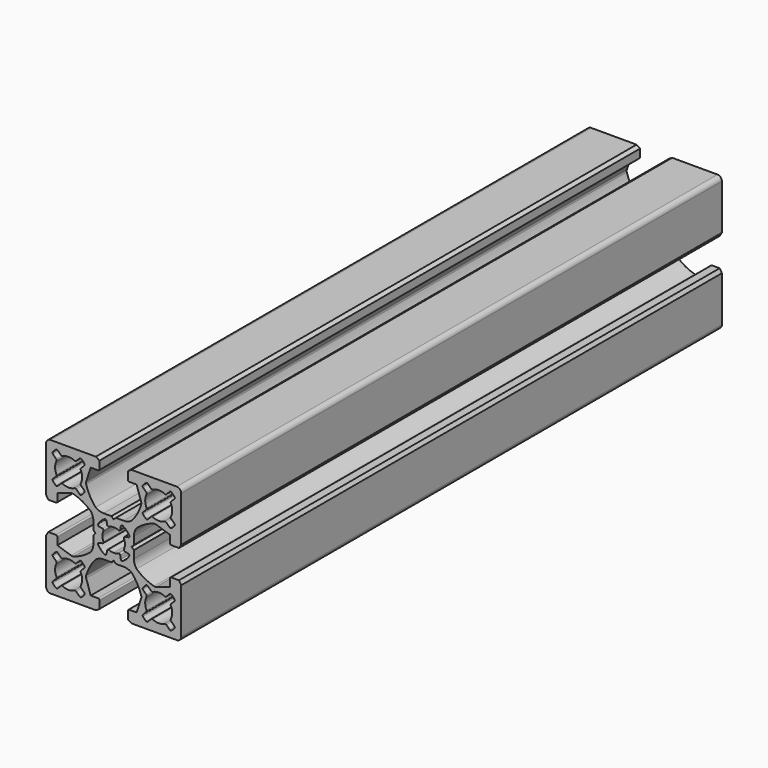
from build123d import *

# Parameters (mm, degrees)
F1_DEPTH = 150


# Not quite as in the source:
# - ends of sketch curves that miss each other by under 0.0002 mm in the source are joined


with BuildPart() as f1:
    # F0 (on Front) → F1 (new body)
    with BuildSketch(Plane.XZ):
        with BuildLine():
            Line((-10.317882, -28.053804), (-8.817882, -28.053804))
            Line((-8.817882, -28.053804), (-8.317882, -27.553804))
            Line((-8.317882, -27.553804), (-8.317882, -25.835963))
            ThreePointArc((-8.317882, -25.835963), (-8.1666472628, -24.8954650055), (-7.7281910149, -24.049790989))
            ThreePointArc((-7.7281910149, -24.049790989), (-5.9278016138, -22.7791417483), (-3.8900220756, -21.9404487353))
            ThreePointArc((-3.8900220756, -21.9404487353), (-3.6281322729, -21.9188378518), (-3.3696549943, -21.9661959825))
            Line((-3.3696549943, -21.9661959825), (-0.317882, -22.953804))
            Line((-0.317882, -22.953804), (-0.317882, -24.603804))
            ThreePointArc((-0.317882, -24.603804), (-0.2300140344, -24.8159360344), (-0.017882, -24.903804))
            Line((-0.017882, -24.903804), (1.682118, -24.903804))
            Line((1.682118, -24.903804), (2.182118, -24.103804))
            Line((2.182118, -24.103804), (2.182118, -14.053804))
            ThreePointArc((2.182118, -14.053804), (1.8892247812, -13.3466972188), (1.182118, -13.053804))
            Line((1.182118, -13.053804), (-8.867882, -13.053804))
            Line((-8.867882, -13.053804), (-9.667882, -13.553804))
            Line((-9.667882, -13.553804), (-9.667882, -15.253804))
            ThreePointArc((-9.667882, -15.253804), (-9.5800140344, -15.4659360344), (-9.367882, -15.553804))
            Line((-9.367882, -15.553804), (-7.717882, -15.553804))
            Line((-7.717882, -15.553804), (-6.730274, -18.605577))
            ThreePointArc((-6.730274, -18.605577), (-6.6829159047, -18.8640542036), (-6.7045263914, -19.1259439149))
            ThreePointArc((-6.7045263914, -19.1259439149), (-7.5432189083, -21.1637239049), (-8.8138685119, -22.9641134339))
            ThreePointArc((-8.8138685119, -22.9641134339), (-9.6595430055, -23.4025692628), (-10.600041, -23.553804))
            Line((-10.600041, -23.553804), (-12.317882, -23.553804))
            Line((-12.317882, -23.553804), (-12.817882, -24.053804))
            Line((-12.817882, -24.053804), (-12.817882, -25.553804))
            ThreePointArc((-12.817882, -25.553804), (-12.2892723342, -25.6103286428), (-11.7845662465, -25.777346543))
            ThreePointArc((-11.7845662465, -25.777346543), (-11.521192295, -25.7698304515), (-11.3653270693, -25.5573959875))
            Line((-11.3653270693, -25.5573959875), (-11.231756, -24.816462))
            ThreePointArc((-11.231756, -24.816462), (-11.061392872, -24.5969122529), (-10.7838767336, -24.6114195492))
            ThreePointArc((-10.7838767336, -24.6114195492), (-9.990624391, -25.2265473595), (-9.3754974572, -26.0198002702))
            ThreePointArc((-9.3754974572, -26.0198002702), (-9.3609903588, -26.2973161033), (-9.5805400125, -26.4676789307))
            Line((-9.5805400125, -26.4676789307), (-10.321473, -26.601249))
            ThreePointArc((-10.321473, -26.601249), (-10.5339073555, -26.757114112), (-10.5414238716, -27.0204879417))
            ThreePointArc((-10.5414238716, -27.0204879417), (-10.3744066428, -27.5251943342), (-10.317882, -28.053804))
        make_face()
        with BuildLine():
            ThreePointArc((-5.5627339656, -19.7356560344), (-5.4787894201, -19.5718836819), (-5.5062620121, -19.389913006))
            ThreePointArc((-5.5062620121, -19.389913006), (-5.820221, -18.053804), (-5.5062614757, -16.7176952608))
            ThreePointArc((-5.5062614757, -16.7176952608), (-5.4787894201, -16.5357243181), (-5.5627339656, -16.3719519656))
            Line((-5.5627339656, -16.3719519656), (-6.303305, -15.631381))
            ThreePointArc((-6.303305, -15.631381), (-6.3907399595, -15.4353436467), (-6.3248118511, -15.2310671199))
            ThreePointArc((-6.3248118511, -15.2310671199), (-6.0022020125, -14.8718239818), (-5.6429589383, -14.5492140766))
            ThreePointArc((-5.6429589383, -14.5492140766), (-5.4386817022, -14.4832850218), (-5.2426439656, -14.5707209656))
            Line((-5.2426439656, -14.5707209656), (-4.502074, -15.311292))
            ThreePointArc((-4.502074, -15.311292), (-4.3383016819, -15.3952365799), (-4.156331006, -15.3677639879))
            ThreePointArc((-4.156331006, -15.3677639879), (-2.8202214477, -15.053804), (-1.484111862, -15.3677637227))
            ThreePointArc((-1.484111862, -15.3677637227), (-1.3021413181, -15.3952365799), (-1.1383689656, -15.3112920344))
            Line((-1.1383689656, -15.3112920344), (-0.397799, -14.570721))
            ThreePointArc((-0.397799, -14.570721), (-0.2017612978, -14.4832850218), (0.0025159751, -14.5492140309))
            ThreePointArc((0.0025159751, -14.5492140309), (0.3617595153, -14.8718234847), (0.684369412, -15.2310666682))
            ThreePointArc((0.684369412, -15.2310666682), (0.7502979573, -15.4353436866), (0.6628620344, -15.6313810344))
            Line((0.6628620344, -15.6313810344), (-0.077709, -16.371952))
            ThreePointArc((-0.077709, -16.371952), (-0.1616535799, -16.5357243181), (-0.1341809879, -16.717694994))
            ThreePointArc((-0.1341809879, -16.717694994), (0.179779, -18.053804), (-0.1341807227, -19.389913138))
            ThreePointArc((-0.1341807227, -19.389913138), (-0.1616535799, -19.5718836819), (-0.0777090344, -19.7356560344))
            Line((-0.0777090344, -19.7356560344), (0.662862, -20.476227))
            ThreePointArc((0.662862, -20.476227), (0.7502979573, -20.6722643134), (0.6843694576, -20.8765413686))
            ThreePointArc((0.6843694576, -20.8765413686), (0.3617595153, -21.2357845153), (0.0025163318, -21.558394412))
            ThreePointArc((0.0025163318, -21.558394412), (-0.2017612978, -21.6243229782), (-0.3977990344, -21.5368870344))
            Line((-0.3977990344, -21.5368870344), (-1.138369, -20.796316))
            ThreePointArc((-1.138369, -20.796316), (-1.3021413181, -20.7123714201), (-1.484111994, -20.7398440121))
            ThreePointArc((-1.484111994, -20.7398440121), (-2.8202214477, -21.053804), (-4.1563309396, -20.7398438786))
            ThreePointArc((-4.1563309396, -20.7398438786), (-4.3383016819, -20.7123714201), (-4.5020740344, -20.7963159656))
            Line((-4.5020740344, -20.7963159656), (-5.242644, -21.536887))
            ThreePointArc((-5.242644, -21.536887), (-5.4386817022, -21.6243229782), (-5.6429589751, -21.5583939691))
            ThreePointArc((-5.6429589751, -21.5583939691), (-6.0022020125, -21.2357840182), (-6.3248118054, -20.8765408433))
            ThreePointArc((-6.3248118054, -20.8765408433), (-6.3907399595, -20.6722643533), (-6.3033045344, -20.4762274656))
            Line((-6.3033045344, -20.4762274656), (-5.5627339656, -19.7356560344))
        make_face(mode=Mode.SUBTRACT)
        with BuildLine():
            Line((-16.817882, -28.053804), (-15.317882, -28.053804))
            ThreePointArc((-15.317882, -28.053804), (-15.2613573135, -27.5251941322), (-15.0943392862, -27.0204878701))
            ThreePointArc((-15.0943392862, -27.0204878701), (-15.1018556445, -26.757114112), (-15.3142900125, -26.6012490693))
            Line((-15.3142900125, -26.6012490693), (-16.055223, -26.467679))
            ThreePointArc((-16.055223, -26.467679), (-16.2747726412, -26.2973161033), (-16.2602657097, -26.0198001716))
            ThreePointArc((-16.2602657097, -26.0198001716), (-15.6451391247, -25.2265468753), (-14.8518861678, -24.611419716))
            ThreePointArc((-14.8518861678, -24.611419716), (-14.574370128, -24.5969122529), (-14.4040070693, -24.8164620125))
            Line((-14.4040070693, -24.8164620125), (-14.270436, -25.557396))
            ThreePointArc((-14.270436, -25.557396), (-14.114570705, -25.7698304515), (-13.8511966819, -25.7773467007))
            ThreePointArc((-13.8511966819, -25.7773467007), (-13.3464912208, -25.6103285465), (-12.817882, -25.553804))
            Line((-12.817882, -25.553804), (-12.817882, -24.053804))
            Line((-12.817882, -24.053804), (-13.317882, -23.553804))
            Line((-13.317882, -23.553804), (-15.035723, -23.553804))
            ThreePointArc((-15.035723, -23.553804), (-15.9762206131, -23.4025693887), (-16.8218943655, -22.9641134932))
            ThreePointArc((-16.8218943655, -22.9641134932), (-18.0925440917, -21.1637239049), (-18.9312372647, -19.1259440756))
            ThreePointArc((-18.9312372647, -19.1259440756), (-18.952848093, -18.864054156), (-18.9054896298, -18.6055767962))
            Line((-18.9054896298, -18.6055767962), (-17.917882, -15.553804))
            Line((-17.917882, -15.553804), (-16.267882, -15.553804))
            ThreePointArc((-16.267882, -15.553804), (-16.0557499656, -15.4659360344), (-15.967882, -15.253804))
            Line((-15.967882, -15.253804), (-15.967882, -13.553804))
            Line((-15.967882, -13.553804), (-16.767882, -13.053804))
            Line((-16.767882, -13.053804), (-26.817882, -13.053804))
            ThreePointArc((-26.817882, -13.053804), (-27.5249887812, -13.3466972188), (-27.817882, -14.053804))
            Line((-27.817882, -14.053804), (-27.817882, -24.103804))
            Line((-27.817882, -24.103804), (-27.317882, -24.903804))
            Line((-27.317882, -24.903804), (-25.617882, -24.903804))
            ThreePointArc((-25.617882, -24.903804), (-25.4057499656, -24.8159360344), (-25.317882, -24.603804))
            Line((-25.317882, -24.603804), (-25.317882, -22.953804))
            Line((-25.317882, -22.953804), (-22.266108, -21.966196))
            ThreePointArc((-22.266108, -21.966196), (-22.0076307271, -21.9188378518), (-21.7457409226, -21.9404486442))
            ThreePointArc((-21.7457409226, -21.9404486442), (-19.7079616374, -22.7791421598), (-17.907572504, -24.049791567))
            ThreePointArc((-17.907572504, -24.049791567), (-17.4691166439, -24.8954652882), (-17.317882, -25.835963))
            Line((-17.317882, -25.835963), (-17.317882, -27.553804))
            Line((-17.317882, -27.553804), (-16.817882, -28.053804))
        make_face()
        with BuildLine():
            ThreePointArc((-20.1318415243, -16.7176952608), (-19.817882, -18.053804), (-20.1318415243, -19.3899127392))
            ThreePointArc((-20.1318415243, -19.3899127392), (-20.1593135799, -19.5718836819), (-20.0753690344, -19.7356560344))
            Line((-20.0753690344, -19.7356560344), (-19.334799, -20.476227))
            ThreePointArc((-19.334799, -20.476227), (-19.2473630595, -20.6722640002), (-19.3132911489, -20.8765408801))
            ThreePointArc((-19.3132911489, -20.8765408801), (-19.6359009875, -21.2357840182), (-19.9951440617, -21.5583939234))
            ThreePointArc((-19.9951440617, -21.5583939234), (-20.1994212978, -21.6243229782), (-20.3954590344, -21.5368870344))
            Line((-20.3954590344, -21.5368870344), (-21.136029, -20.796316))
            ThreePointArc((-21.136029, -20.796316), (-21.2998015274, -20.7123715492), (-21.4817721923, -20.7398436134))
            ThreePointArc((-21.4817721923, -20.7398436134), (-22.8178815523, -21.053804), (-24.153991138, -20.7398442773))
            ThreePointArc((-24.153991138, -20.7398442773), (-24.3359616819, -20.7123714201), (-24.4997340344, -20.7963159656))
            Line((-24.4997340344, -20.7963159656), (-25.240304, -21.536887))
            ThreePointArc((-25.240304, -21.536887), (-25.4363417022, -21.6243229782), (-25.6406189751, -21.5583939691))
            ThreePointArc((-25.6406189751, -21.5583939691), (-25.9998625153, -21.2357845153), (-26.322472412, -20.8765413318))
            ThreePointArc((-26.322472412, -20.8765413318), (-26.3884009573, -20.6722643134), (-26.3009650344, -20.4762269656))
            Line((-26.3009650344, -20.4762269656), (-25.560394, -19.735656))
            ThreePointArc((-25.560394, -19.735656), (-25.4764494201, -19.5718836819), (-25.5039220121, -19.389913006))
            ThreePointArc((-25.5039220121, -19.389913006), (-25.817882, -18.053804), (-25.5039222773, -16.717694862))
            ThreePointArc((-25.5039222773, -16.717694862), (-25.4764494201, -16.5357243181), (-25.5603939656, -16.3719519656))
            Line((-25.5603939656, -16.3719519656), (-26.300965, -15.631381))
            ThreePointArc((-26.300965, -15.631381), (-26.3884009573, -15.4353436866), (-26.3224724576, -15.2310666314))
            ThreePointArc((-26.3224724576, -15.2310666314), (-25.9998625153, -14.8718234847), (-25.6406193318, -14.549213588))
            ThreePointArc((-25.6406193318, -14.549213588), (-25.4363417022, -14.4832850218), (-25.2403039656, -14.5707209656))
            Line((-25.2403039656, -14.5707209656), (-24.499734, -15.311292))
            ThreePointArc((-24.499734, -15.311292), (-24.3359616819, -15.3952365799), (-24.153991006, -15.3677639879))
            ThreePointArc((-24.153991006, -15.3677639879), (-22.8178815523, -15.053804), (-21.4817720604, -15.3677641214))
            ThreePointArc((-21.4817720604, -15.3677641214), (-21.2998015274, -15.3952364508), (-21.1360294656, -15.3112915344))
            Line((-21.1360294656, -15.3112915344), (-20.395459, -14.570721))
            ThreePointArc((-20.395459, -14.570721), (-20.1994212978, -14.4832850218), (-19.9951440249, -14.5492140309))
            ThreePointArc((-19.9951440249, -14.5492140309), (-19.6359009875, -14.8718239818), (-19.3132911946, -15.2310671567))
            ThreePointArc((-19.3132911946, -15.2310671567), (-19.2473630595, -15.4353439998), (-19.3347989656, -15.6313810344))
            Line((-19.3347989656, -15.6313810344), (-20.075369, -16.371952))
            ThreePointArc((-20.075369, -16.371952), (-20.1593135799, -16.5357243181), (-20.1318415243, -16.7176952608))
        make_face(mode=Mode.SUBTRACT)
        with BuildLine():
            ThreePointArc((-15.0943392862, -29.0871201299), (-15.2613573135, -28.5824138678), (-15.317882, -28.053804))
            Line((-15.317882, -28.053804), (-16.817882, -28.053804))
            Line((-16.817882, -28.053804), (-17.317882, -28.553804))
            Line((-17.317882, -28.553804), (-17.317882, -30.271645))
            ThreePointArc((-17.317882, -30.271645), (-17.4691166439, -31.2121427118), (-17.9075726307, -32.0578165326))
            ThreePointArc((-17.9075726307, -32.0578165326), (-19.7079616374, -33.3284658402), (-21.7457409999, -34.1671590005))
            ThreePointArc((-21.7457409999, -34.1671590005), (-22.0076307271, -34.1887701482), (-22.2661080057, -34.1414120175))
            Line((-22.2661080057, -34.1414120175), (-25.317882, -33.153804))
            Line((-25.317882, -33.153804), (-25.317882, -31.503804))
            ThreePointArc((-25.317882, -31.503804), (-25.4057499656, -31.2916719656), (-25.617882, -31.203804))
            Line((-25.617882, -31.203804), (-27.317882, -31.203804))
            Line((-27.317882, -31.203804), (-27.817882, -32.003804))
            Line((-27.817882, -32.003804), (-27.817882, -42.053804))
            ThreePointArc((-27.817882, -42.053804), (-27.5249887812, -42.7609107812), (-26.817882, -43.053804))
            Line((-26.817882, -43.053804), (-16.767882, -43.053804))
            Line((-16.767882, -43.053804), (-15.967882, -42.553804))
            Line((-15.967882, -42.553804), (-15.967882, -40.853804))
            ThreePointArc((-15.967882, -40.853804), (-16.0557499656, -40.6416719656), (-16.267882, -40.553804))
            Line((-16.267882, -40.553804), (-17.917882, -40.553804))
            Line((-17.917882, -40.553804), (-18.905489, -37.50203))
            ThreePointArc((-18.905489, -37.50203), (-18.9528481165, -37.2435533689), (-18.9312375634, -36.9816638775))
            ThreePointArc((-18.9312375634, -36.9816638775), (-18.0925440917, -34.9438840951), (-16.8218944881, -33.1434945661))
            ThreePointArc((-16.8218944881, -33.1434945661), (-15.9762206131, -32.7050386113), (-15.035723, -32.553804))
            Line((-15.035723, -32.553804), (-13.317882, -32.553804))
            Line((-13.317882, -32.553804), (-12.817882, -32.053804))
            Line((-12.817882, -32.053804), (-12.817882, -30.553804))
            ThreePointArc((-12.817882, -30.553804), (-13.3464914228, -30.4972794098), (-13.8511973007, -30.3302616625))
            ThreePointArc((-13.8511973007, -30.3302616625), (-14.114570888, -30.3377776445), (-14.2704359307, -30.5502120125))
            Line((-14.2704359307, -30.5502120125), (-14.404007, -31.291146))
            ThreePointArc((-14.404007, -31.291146), (-14.574370128, -31.5106957471), (-14.8518862664, -31.4961884508))
            ThreePointArc((-14.8518862664, -31.4961884508), (-15.6451391247, -30.8810611247), (-16.260266284, -30.0878081678))
            ThreePointArc((-16.260266284, -30.0878081678), (-16.2747726412, -29.8102918967), (-16.0552229875, -29.6399290693))
            Line((-16.0552229875, -29.6399290693), (-15.31429, -29.506358))
            ThreePointArc((-15.31429, -29.506358), (-15.1018556033, -29.3504938095), (-15.0943392862, -29.0871201299))
        make_face()
        with BuildLine():
            ThreePointArc((-20.0747205338, -36.3725174663), (-20.1586523342, -36.5362963089), (-20.1311656295, -36.7182648157))
            ThreePointArc((-20.1311656295, -36.7182648157), (-19.8171020091, -38.0543498837), (-20.1309575628, -39.3904837201))
            ThreePointArc((-20.1309575628, -39.3904837201), (-20.1584156946, -39.5724564631), (-20.0744580337, -39.7362220337))
            Line((-20.0744580337, -39.7362220337), (-19.33383, -40.476735))
            ThreePointArc((-19.33383, -40.476735), (-19.2463783169, -40.6727656131), (-19.3122908476, -40.8770481227))
            ThreePointArc((-19.3122908476, -40.8770481227), (-19.6348730769, -41.2363160882), (-19.9940910142, -41.5589539824))
            ThreePointArc((-19.9940910142, -41.5589539824), (-20.1983629105, -41.6248982338), (-20.3944070337, -41.5374780337))
            Line((-20.3944070337, -41.5374780337), (-21.135036, -40.796965))
            ThreePointArc((-21.135036, -40.796965), (-21.2988146578, -40.7130336089), (-21.4807828157, -40.7405203705))
            ThreePointArc((-21.4807828157, -40.7405203705), (-22.8168676587, -41.0545839908), (-24.1530013171, -40.7407286377))
            ThreePointArc((-24.1530013171, -40.7407286377), (-24.334973892, -40.7132702121), (-24.4987395337, -40.7972274662))
            Line((-24.4987395337, -40.7972274662), (-25.239253, -41.537856))
            ThreePointArc((-25.239253, -41.537856), (-25.435283708, -41.625306742), (-25.6395657293, -41.5593936639))
            ThreePointArc((-25.6395657293, -41.5593936639), (-25.99883431, -41.2368127014), (-26.3214719824, -40.8775949858))
            ThreePointArc((-26.3214719824, -40.8775949858), (-26.3874162149, -40.6733227364), (-26.2999955337, -40.4772784662))
            Line((-26.2999955337, -40.4772784662), (-25.559483, -39.73665))
            ThreePointArc((-25.559483, -39.73665), (-25.475550759, -39.5728712621), (-25.5030371701, -39.3909025871))
            ThreePointArc((-25.5030371701, -39.3909025871), (-25.8171019909, -38.0548178936), (-25.503246239, -36.7186838812))
            ThreePointArc((-25.503246239, -36.7186838812), (-25.4757871762, -36.5367113277), (-25.5597444663, -36.3729454662))
            Line((-25.5597444663, -36.3729454662), (-26.300374, -35.632433))
            ThreePointArc((-26.300374, -35.632433), (-26.3878247021, -35.4364020339), (-26.3219121524, -35.2321198773))
            ThreePointArc((-26.3219121524, -35.2321198773), (-25.9993304261, -34.8728514147), (-25.6401123794, -34.550213529))
            ThreePointArc((-25.6401123794, -34.550213529), (-25.4358403078, -34.4842688081), (-25.2397959662, -34.5716899662))
            Line((-25.2397959662, -34.5716899662), (-24.499168, -35.312203))
            ThreePointArc((-24.499168, -35.312203), (-24.3353886912, -35.3961343342), (-24.1534201843, -35.3686476295))
            ThreePointArc((-24.1534201843, -35.3686476295), (-22.8173356686, -35.0545840091), (-21.4812022799, -35.3684395628))
            ThreePointArc((-21.4812022799, -35.3684395628), (-21.2992289788, -35.3958977668), (-21.1354629663, -35.3119400337))
            Line((-21.1354629663, -35.3119400337), (-20.39495, -34.571312))
            ThreePointArc((-20.39495, -34.571312), (-20.1989200339, -34.4838602979), (-19.9946378773, -34.5497728476))
            ThreePointArc((-19.9946378773, -34.5497728476), (-19.63536969, -34.8723552987), (-19.312731624, -35.2315735027))
            ThreePointArc((-19.312731624, -35.2315735027), (-19.2467867662, -35.4358449105), (-19.3342069663, -35.6318890337))
            Line((-19.3342069663, -35.6318890337), (-20.0747205338, -36.3725174663))
        make_face(mode=Mode.SUBTRACT)
        with BuildLine():
            Line((-8.317882, -28.553804), (-8.817882, -28.053804))
            Line((-8.817882, -28.053804), (-10.317882, -28.053804))
            ThreePointArc((-10.317882, -28.053804), (-10.3744066428, -28.5824136658), (-10.541424543, -29.0871197535))
            ThreePointArc((-10.541424543, -29.0871197535), (-10.5339073967, -29.3504938095), (-10.3214731621, -29.5063588992))
            Line((-10.3214731621, -29.5063588992), (-9.58054, -29.639929))
            ThreePointArc((-9.58054, -29.639929), (-9.3609903588, -29.8102918967), (-9.3754972903, -30.0878078284))
            ThreePointArc((-9.3754972903, -30.0878078284), (-9.990624391, -30.8810606405), (-10.783877091, -31.496187846))
            ThreePointArc((-10.783877091, -31.496187846), (-11.061392872, -31.5106957471), (-11.2317559307, -31.2911459875))
            Line((-11.2317559307, -31.2911459875), (-11.365327, -30.550212))
            ThreePointArc((-11.365327, -30.550212), (-11.521192112, -30.3377776445), (-11.7845659417, -30.3302611284))
            ThreePointArc((-11.7845659417, -30.3302611284), (-12.2892721322, -30.4972793135), (-12.817882, -30.553804))
            Line((-12.817882, -30.553804), (-12.817882, -32.053804))
            Line((-12.817882, -32.053804), (-12.317882, -32.553804))
            Line((-12.317882, -32.553804), (-10.600041, -32.553804))
            ThreePointArc((-10.600041, -32.553804), (-9.6595430055, -32.7050387372), (-8.813868989, -33.1434949851))
            ThreePointArc((-8.813868989, -33.1434949851), (-7.5432189083, -34.9438840951), (-6.7045257353, -36.9816639244))
            ThreePointArc((-6.7045257353, -36.9816639244), (-6.6829158812, -37.2435533212), (-6.7302739825, -37.5020300057))
            Line((-6.7302739825, -37.5020300057), (-7.717882, -40.553804))
            Line((-7.717882, -40.553804), (-9.367882, -40.553804))
            ThreePointArc((-9.367882, -40.553804), (-9.5800140344, -40.6416719656), (-9.667882, -40.853804))
            Line((-9.667882, -40.853804), (-9.667882, -42.553804))
            Line((-9.667882, -42.553804), (-8.867882, -43.053804))
            Line((-8.867882, -43.053804), (1.182118, -43.053804))
            ThreePointArc((1.182118, -43.053804), (1.8892247812, -42.7609107812), (2.182118, -42.053804))
            Line((2.182118, -42.053804), (2.182118, -32.003804))
            Line((2.182118, -32.003804), (1.682118, -31.203804))
            Line((1.682118, -31.203804), (-0.017882, -31.203804))
            ThreePointArc((-0.017882, -31.203804), (-0.2300140344, -31.2916719656), (-0.317882, -31.503804))
            Line((-0.317882, -31.503804), (-0.317882, -33.153804))
            Line((-0.317882, -33.153804), (-3.369655, -34.141412))
            ThreePointArc((-3.369655, -34.141412), (-3.6281322729, -34.1887701482), (-3.8900220774, -34.1671593558))
            ThreePointArc((-3.8900220774, -34.1671593558), (-5.9278016138, -33.3284662517), (-7.7281909374, -32.0578169295))
            ThreePointArc((-7.7281909374, -32.0578169295), (-8.1666472628, -31.2121429945), (-8.317882, -30.271645))
            Line((-8.317882, -30.271645), (-8.317882, -28.553804))
        make_face()
        with BuildLine():
            ThreePointArc((-5.507146239, -39.3904841188), (-5.8210019909, -38.0543501064), (-5.5069379006, -36.7182650494))
            ThreePointArc((-5.5069379006, -36.7182650494), (-5.4794506299, -36.5362965287), (-5.5633824662, -36.3725174663))
            Line((-5.5633824662, -36.3725174663), (-6.303896, -35.631889))
            ThreePointArc((-6.303896, -35.631889), (-6.3913162338, -35.4358449105), (-6.3253716664, -35.2315732687))
            ThreePointArc((-6.3253716664, -35.2315732687), (-6.0027340882, -34.8723550769), (-5.6434657786, -34.5497732749))
            ThreePointArc((-5.6434657786, -34.5497732749), (-5.4391833549, -34.483860277), (-5.2431524662, -34.5713114663))
            Line((-5.2431524662, -34.5713114663), (-4.50264, -35.31194))
            ThreePointArc((-4.50264, -35.31194), (-4.3388740212, -35.3958977668), (-4.1569008286, -35.3684393446))
            ThreePointArc((-4.1569008286, -35.3684393446), (-2.8207674361, -35.0545840092), (-1.4846830494, -35.3686480994))
            ThreePointArc((-1.4846830494, -35.3686480994), (-1.3027146578, -35.3961343911), (-1.1389359663, -35.3122030337))
            Line((-1.1389359663, -35.3122030337), (-0.398307, -34.57169))
            ThreePointArc((-0.398307, -34.57169), (-0.2022626922, -34.4842688081), (0.0020096134, -34.5502132386))
            ThreePointArc((0.0020096134, -34.5502132386), (0.3612269231, -34.8728519118), (0.6838087251, -35.2321202214))
            ThreePointArc((0.6838087251, -35.2321202214), (0.7497216831, -35.4364023869), (0.6622700337, -35.6324330337))
            Line((0.6622700337, -35.6324330337), (-0.078358, -36.372946))
            ThreePointArc((-0.078358, -36.372946), (-0.1623158238, -36.5367113277), (-0.1348573446, -36.7186841714))
            ThreePointArc((-0.1348573446, -36.7186841714), (0.1789979909, -38.0548178935), (-0.1350659009, -39.3909025518))
            ThreePointArc((-0.1350659009, -39.3909025518), (-0.162552241, -39.5728712621), (-0.0786200338, -39.7366500338))
            Line((-0.0786200338, -39.7366500338), (0.661893, -40.477278))
            ThreePointArc((0.661893, -40.477278), (0.7493132149, -40.6733227364), (0.6833686664, -40.8775947313))
            ThreePointArc((0.6833686664, -40.8775947313), (0.3607308072, -41.2368122042), (0.0014628737, -41.5593938432))
            ThreePointArc((0.0014628737, -41.5593938432), (-0.202819292, -41.625306742), (-0.3988500338, -41.5378560338))
            Line((-0.3988500338, -41.5378560338), (-1.139363, -40.797227))
            ThreePointArc((-1.139363, -40.797227), (-1.303129108, -40.7132702121), (-1.4851017727, -40.7407284571))
            ThreePointArc((-1.4851017727, -40.7407284571), (-2.8212354459, -41.0545839909), (-4.157320149, -40.7405202994))
            ThreePointArc((-4.157320149, -40.7405202994), (-4.3392886912, -40.7130336658), (-4.5030675338, -40.7969654663))
            Line((-4.5030675338, -40.7969654663), (-5.243696, -41.537478))
            ThreePointArc((-5.243696, -41.537478), (-5.4397403476, -41.624898194), (-5.6440121248, -41.5589541549))
            ThreePointArc((-5.6440121248, -41.5589541549), (-6.0032304261, -41.2363165853), (-6.3258123317, -40.8770482671))
            ThreePointArc((-6.3258123317, -40.8770482671), (-6.3917246831, -40.6727656131), (-6.3042730337, -40.4767349663))
            Line((-6.3042730337, -40.4767349663), (-5.563645, -39.736222))
            ThreePointArc((-5.563645, -39.736222), (-5.4796873054, -39.5724564631), (-5.507146239, -39.3904841188))
        make_face(mode=Mode.SUBTRACT)
    extrude(amount=F1_DEPTH)


solid = f1.part
